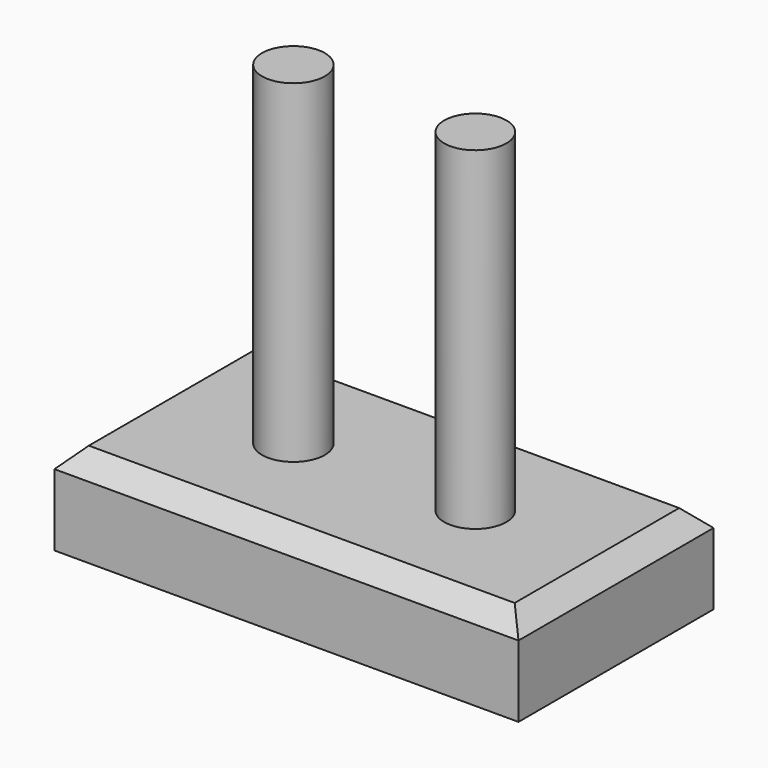
from build123d import *

# Parameters (mm, degrees)
F0_W         = 123.3936399221
F0_H         = 64.8306235671
F1_DEPTH     = 24.13
F2_SIZE      = 5.08
F3_W         = 43.4815697372
F3_H         = 12.9269515164
F4_DEPTH     = 2.54
F5_TEXT_SIZE = 4.3525101824
F6_DEPTH     = 1.524
F7_R         = 8.2733248393
F7_R_2       = 8.3609613394
F8_DEPTH     = 112.776


# Not quite as in the source:
# - Text() gives the source's letters only with a copy of the font that has no kerning and outlines rounded to 1/6400 em; it was checked with that copy


with BuildPart() as f1:
    # F0 (on Top) → F1 (new body)
    with BuildSketch(Plane.XY):
        Rectangle(F0_W, F0_H)
    extrude(amount=F1_DEPTH)

    # F2
    f2_edges = [f1.edges().sort_by_distance(p)[0] for p in [
        (0, 32.415312, 24.13),
        (-61.69682, 0, 24.13),
        (0, -32.415312, 24.13),
        (61.69682, 0, 24.13),
    ]]
    chamfer(f2_edges, length=F2_SIZE)

    # F3 (on face) → F4 (join)
    with BuildSketch(Plane(origin=(0, 32.4153117836, 0), x_dir=(-1, 0, 0), z_dir=(0, 1, 0))):
        with Locations((0, 10.2828023955)):
            Rectangle(F3_W, F3_H)
    extrude(amount=F4_DEPTH)

    # F5 (on face) → F6 (join)
    with BuildSketch(Plane(origin=(0, 34.9553117836, 0), x_dir=(-1, 0, 0), z_dir=(0, 1, 0))):
        with Locations((-15.8648956567, 11.4579806104)):
            Text('Rezwan Rahman', F5_TEXT_SIZE, font='Open Sans', text_align=(TextAlign.LEFT, TextAlign.BOTTOM))
    extrude(amount=F6_DEPTH)

    # F7 (on face) → F8 (join)
    with BuildSketch(Plane(origin=(0, 0, 0), x_dir=(1, 0, 0), z_dir=(0, 0, -1))):
        with Locations((24.2870002985, 0)):
            Circle(F7_R)
        with Locations((-24.0911394358, 0)):
            Circle(F7_R_2)
    extrude(amount=-F8_DEPTH)


solid = f1.part
